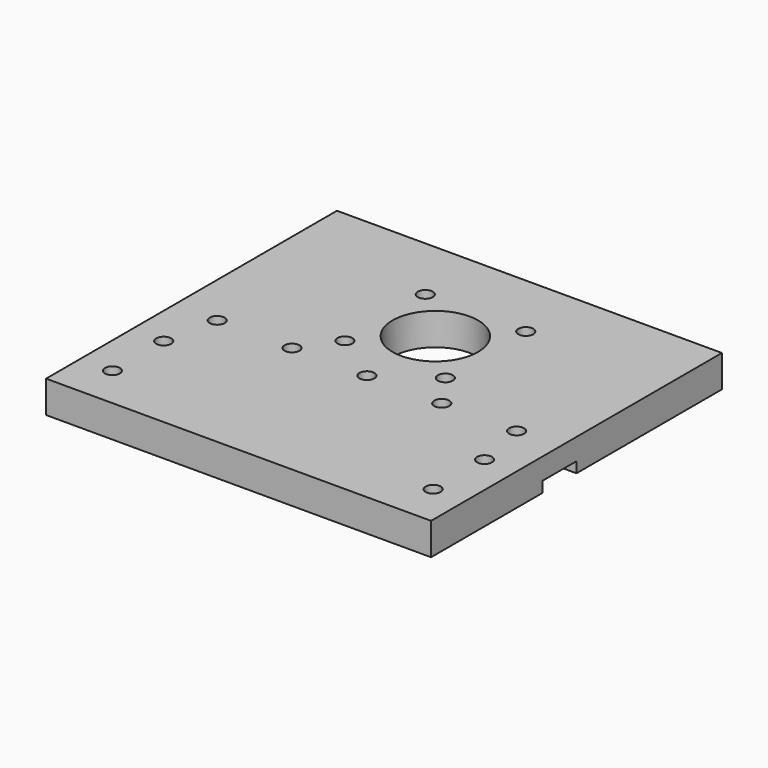
from build123d import *

# Parameters (mm, degrees)
F0_W      = 170
F0_H      = 15
F1_DEPTH  = 150
F2_W      = 170
F2_H      = 20
F3_DEPTH  = 5
F4_R      = 20
F5_DEPTH  = 25
F7_D      = 7
F8_DEPTH  = 5
F9_DEPTH  = 5
F11_D     = 7
F13_D     = 7
F14_DEPTH = 20
F16_D     = 7


# Not quite as in the source:
# - a feature names something its author has since deleted; it is built from what else it names


with BuildPart() as f1:
    # F0 (on Front) → F1 (new body)
    with BuildSketch(Plane.XZ):
        with Locations((85, 7.5)):
            Rectangle(F0_W, F0_H)
    extrude(amount=F1_DEPTH)

    # F2 (on face) → F3 (cut)
    with BuildSketch(Plane(origin=(0, 0, 0), x_dir=(1, 0, 0), z_dir=(0, 0, -1))):
        with Locations((85, 95)):
            Rectangle(F2_W, F2_H)
    extrude(amount=-F3_DEPTH, mode=Mode.SUBTRACT)

    # F4 (on face) → F5 (cut)
    with BuildSketch(Plane.XY.offset(15)):
        with Locations((85, -55)):
            Circle(F4_R)
    extrude(amount=-F5_DEPTH, mode=Mode.SUBTRACT)

    # F7 (through all)
    with Locations(Plane.XY.offset(15)):
        with Locations((61.5, -31.5), (61.5, -78.5), (108.5, -78.5), (108.5, -31.5)):
            Hole(F7_D / 2)

    # F8 (add): a face of the model
    f8_faces = [f1.faces().sort_by_distance(p)[0] for p in [
        (0, -74.0697674419, 7.7325581395),
    ]]
    extrude(f8_faces, amount=F8_DEPTH)

    # F9 (add): a face of the model
    f9_faces = [f1.faces().sort_by_distance(p)[0] for p in [
        (170, -74.0697674419, 7.7325581395),
    ]]
    extrude(f9_faces, amount=F9_DEPTH)

    # F11 (through all)
    with Locations(Plane.XY.offset(15)):
        with Locations((50, -95), (15, -95), (85, -95), (120, -95), (155, -95)):
            Hole(F11_D / 2)

    # F13 (through all)
    with Locations(Plane.XY.offset(15)):
        with Locations((10, -120), (160, -120)):
            Hole(F13_D / 2)

    # F14 (add): a face of the model
    f14_faces = [f1.faces().sort_by_distance(p)[0] for p in [
        (85, -150, 7.5),
    ]]
    extrude(f14_faces, amount=F14_DEPTH)

    # F16 (through all)
    with Locations(Plane.XY.offset(15)):
        with Locations((10, -150), (160, -150)):
            Hole(F16_D / 2)


solid = f1.part
